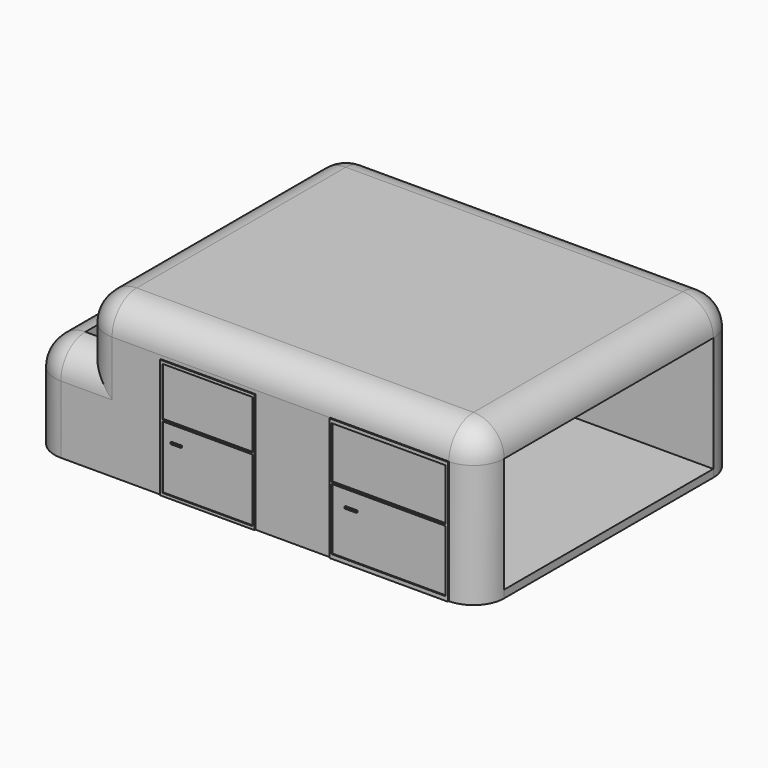
from build123d import *

# Parameters (mm, degrees)
F0_W      = 65.8210366964
F0_H      = 53.360377121
F1_DEPTH  = 25.4
F0_W_2    = 8.4739662707
F2_DEPTH  = 16.256
F3_R      = 5.08
F4_R      = 5.08
F6_W      = 14.9103230797
F6_H      = 10.4163230571
F6_H_2    = 8.0820930889
F6_W_2    = 1.7418600619
F6_H_3    = 0.2754591405
F8_DEPTH  = 0.1778
F6_W_3    = 18.7708195299
F6_H_4    = 10.2186049917
F6_H_5    = 8.557209163
F6_W_4    = 1.9885748625
F9_DEPTH  = 0.2032
F10_W     = 1.7440356314
F10_H     = 0.2743424848
F11_DEPTH = 0.2032
F7_W      = 43.200377121
F7_H      = 4.064
F12_DEPTH = 66.04
F13_DEPTH = 14.986


# Not quite as in the source:
# - two fillets or chamfers of one size are made in one step


with BuildPart() as f1:
    # F0 (on Top) → F1 (new body)
    with BuildSketch(Plane.XY):
        Rectangle(F0_W, F0_H)
    extrude(amount=F1_DEPTH)

    # F0 (on Top) → F2 (join)
    with BuildSketch(Plane.XY):
        with Locations((-37.1475014836, 0)):
            Rectangle(F0_W_2, F0_H)
    extrude(amount=F2_DEPTH)

    # F3
    f3_edges = [f1.edges().sort_by_distance(p)[0] for p in [
        (-32.910518, 0, 25.4),
        (-41.384485, 0, 16.256),
    ]]
    fillet(f3_edges, radius=F3_R)

    # F4
    f4_edges = [f1.edges().sort_by_distance(p)[0] for p in [
        (2.54, -26.680189, 25.4),
        (2.54, 26.680189, 25.4),
        (32.910518, 0, 25.4),
        (-39.896587, -26.680189, 14.768102),
        (-39.896587, 26.680189, 14.768102),
        (-32.910518, -26.680189, 18.288),
        (-32.910518, 26.680189, 18.288),
        (-31.422621, -26.680189, 23.912102),
        (-34.607501, -26.680189, 16.256),
        (32.910518, -26.680189, 12.7),
        (-41.384485, -26.680189, 5.588),
        (-31.422621, 26.680189, 23.912102),
        (-34.607501, 26.680189, 16.256),
        (32.910518, 26.680189, 12.7),
        (-41.384485, 26.680189, 5.588),
    ]]
    fillet(f4_edges, radius=F4_R)

    # F6 (on face) → F8 (join)
    with BuildSketch(Plane.XZ.offset(26.6801885605)):
        Polygon((-19.7755768895, 0), (-4.168510437, 0), (-4.168510437, 11.176), (-4.168510437, 19.733209163), (-19.7755768895, 19.733209163), (-19.7755768895, 11.176), align=None)
        with Locations((-11.9322177488, 5.6890027045)):
            Rectangle(F6_W, F6_H, mode=Mode.SUBTRACT)
        with Locations((-11.9322177488, 15.2170465444)):
            Rectangle(F6_W, F6_H_2, mode=Mode.SUBTRACT)
        with Locations((-17.1627867967, 8.1434063613)):
            Rectangle(F6_W_2, F6_H_3)
    extrude(amount=F8_DEPTH)

    # F6 (on face) → F9 (join)
    with BuildSketch(Plane.XZ.offset(26.6801885605)):
        Polygon((8.2342270762, 20.32), (8.2342270762, 11.176), (8.2342270762, 0), (27.8305183482, 0), (27.8305183482, 11.176), (27.8305183482, 19.733209163), (27.8305183482, 20.32), align=None)
        with Locations((18.0146349594, 5.7878617372)):
            Rectangle(F6_W_3, F6_H_4, mode=Mode.SUBTRACT)
        with Locations((18.0146349594, 15.4546045815)):
            Rectangle(F6_W_3, F6_H_5, mode=Mode.SUBTRACT)
        with Locations((11.7142330855, 8.1434063613)):
            Rectangle(F6_W_4, F6_H_3)
    extrude(amount=F9_DEPTH)

    # F10 (on face) → F11 (join)
    with BuildSketch(Plane(origin=(0, 26.6801885605, 0), x_dir=(-1, 0, 0), z_dir=(0, 1, 0))):
        Polygon((-27.8305183482, 0), (-8.2305837423, 0), (-8.2305837423, 10.9018748626), (-8.2305837423, 20.32), (-27.8305183482, 20.32), (-27.8305183482, 11.2858796492), (-27.8305183482, 10.9018748626), align=None)
        Polygon((-8.626322262, 0.6852262607), (-27.4223405868, 0.7035561139), (-27.4223405868, 10.9018748626), (-8.626322262, 10.9018748626), align=None, mode=Mode.SUBTRACT)
        Polygon((-27.3978635669, 11.1784273759), (-27.3978635669, 19.7369996458), (-8.626322262, 19.7369996458), (-8.6272079498, 11.1749703065), align=None, mode=Mode.SUBTRACT)
        Polygon((-10.7196969911, 8.2838209346), (-12.7080604434, 8.287482895), (-12.7080604434, 8.0091850832), (-10.7196969911, 8.0091850832), align=None)
        Polygon((4.1694319807, 10.9128411859), (4.1694319807, 0), (19.7687353939, 0), (19.7687353939, 10.9128411859), (19.7687353939, 11.1958524212), (19.7687353939, 19.7498388588), (4.1547794826, 19.7498388588), (4.1547794826, 11.1958505586), align=None)
        Polygon((4.4739199802, 0.4796771973), (4.4739199802, 10.9128411859), (19.3859692663, 10.8820935711), (19.3859692663, 0.4796771973), align=None, mode=Mode.SUBTRACT)
        Polygon((19.3879064173, 19.2518327385), (19.3879064173, 11.1958524212), (4.4739199802, 11.1958505586), (4.4477242045, 19.2518327385), align=None, mode=Mode.SUBTRACT)
        with Locations((17.162848264, 8.1434589811)):
            Rectangle(F10_W, F10_H)
    extrude(amount=F11_DEPTH)

    # F7 (on face) → F12 (cut)
    with BuildSketch(Plane(origin=(-32.9105183482, 0, 0), x_dir=(0, -1, 0), z_dir=(-1, 0, 0))):
        with Locations((0, 18.288)):
            Rectangle(F7_W, F7_H)
    extrude(amount=-F12_DEPTH, mode=Mode.SUBTRACT)

    # F13 (cut): a face of the model
    f13_faces = [f1.faces().sort_by_distance(p)[0] for p in [
        (-1.6969831353, 0, 16.256),
    ]]
    extrude(f13_faces, amount=-F13_DEPTH, mode=Mode.SUBTRACT)


solid = f1.part
